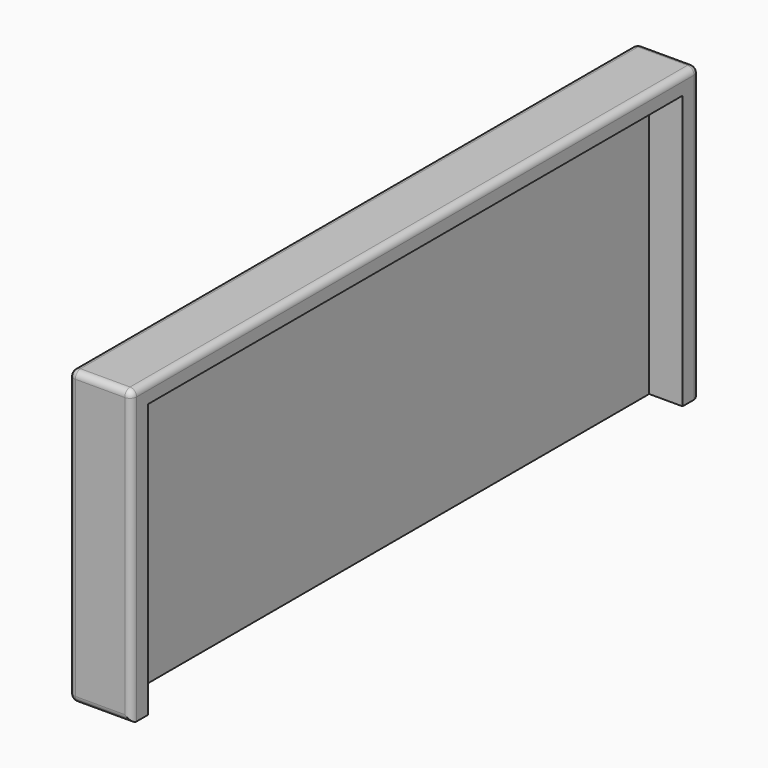
from build123d import *

# Parameters (mm, degrees)
F0_W     = 19.05
F0_H     = 215.9
F1_DEPTH = 88.9
F2_W     = 203.2
F2_H     = 83.2
F3_DEPTH = 10.16
F4_R     = 2


# Not quite as in the source:
# - a feature names something its author has since deleted; it is built from what else it names


with BuildPart() as f1:
    # F0 (on Top) → F1 (new body)
    with BuildSketch(Plane.XY):
        Rectangle(F0_W, F0_H)
    extrude(amount=F1_DEPTH)

    # F2 (on face) → F3 (cut)
    with BuildSketch(Plane.YZ.offset(9.525)):
        with Locations((0, 41.6)):
            Rectangle(F2_W, F2_H)
    extrude(amount=-F3_DEPTH, mode=Mode.SUBTRACT)

    # F4
    f4_edges = [f1.edges().sort_by_distance(p)[0] for p in [
        (-9.525, 0, 88.9),
        (0, -107.95, 88.9),
        (-9.525, -107.95, 44.45),
        (-9.525, 107.95, 44.45),
        (0, 107.95, 88.9),
        (9.525, 0, 88.9),
        (9.525, -107.95, 44.45),
        (9.525, 107.95, 44.45),
        (-9.525, 0, 0),
        (0, 107.95, 0),
        (0, -107.95, 0),
    ]]
    fillet(f4_edges, radius=F4_R)


solid = f1.part
